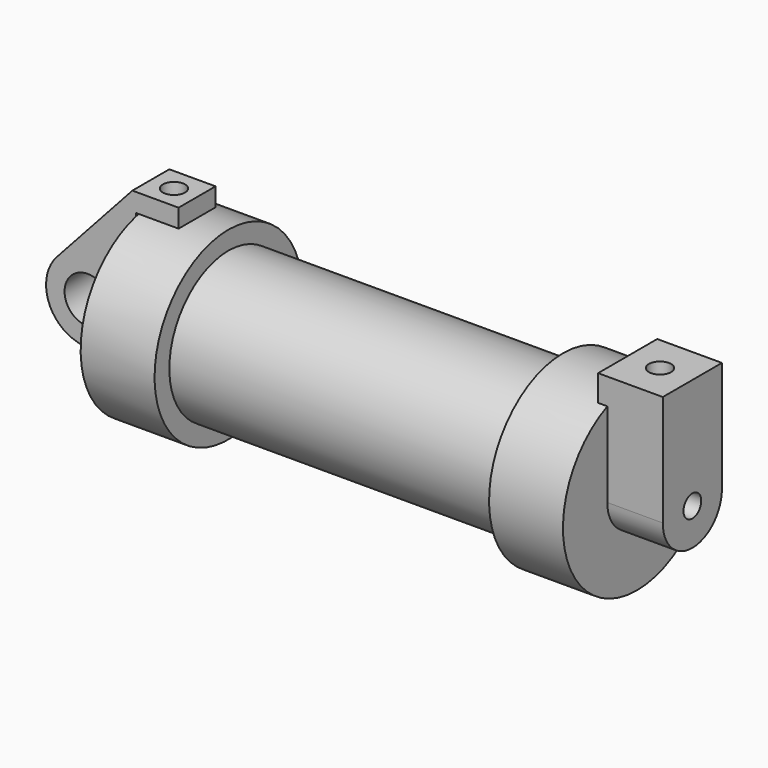
from build123d import *

# Parameters (mm, degrees)
F0_W          = 5.842
F0_H          = 12.7
F0_R          = 3.175
F2_DEPTH      = 3.175
F3_R          = 1.524
F4_DEPTH      = 7.62
F4_DEPTH_BACK = 1.27
F5_R          = 1.524
F6_DEPTH      = 10.414
F7_R          = 1.524
F8_DEPTH      = 17.78


with BuildPart() as f1:
    # F0 (on Front) → F1 (revolve)
    with BuildSketch(Plane.XZ):
        Polygon((5.842, 12.7), (5.842, 0), (66.294, 0), (66.294, 12.7), (56.134, 12.7), (56.134, 10.16), (10.16, 10.16), (10.16, 12.7), align=None)
        with Locations((2.921, 6.35)):
            Rectangle(F0_W, F0_H)
    revolve(axis=Axis((33.147, 0, 0), (-1, 0, 0)))

    # F3 (on face) → F4 (join, two sides)
    with BuildSketch(Plane.YZ.offset(66.294)) as f4_sk:
        with BuildLine():
            ThreePointArc((-5.08, 0), (0, -5.08), (5.08, 0))
            ThreePointArc((5.08, 0), (0, 5.08), (-5.08, 0))
        make_face()
        Circle(F3_R, mode=Mode.SUBTRACT)
        with BuildLine():
            ThreePointArc((-5.08, 11.6397422652), (0, 12.7), (5.08, 11.6397422652))
            Line((5.08, 11.6397422652), (5.08, 15.24))
            Line((5.08, 15.24), (-5.08, 15.24))
            Line((-5.08, 15.24), (-5.08, 11.6397422652))
        make_face()
        with BuildLine():
            ThreePointArc((-5.08, 0), (0, 5.08), (5.08, 0))
            Line((5.08, 0), (5.08, 11.6397422652))
            ThreePointArc((5.08, 11.6397422652), (0, 12.7), (-5.08, 11.6397422652))
            Line((-5.08, 11.6397422652), (-5.08, 0))
        make_face()
    extrude(amount=F4_DEPTH)
    extrude(f4_sk.sketch, amount=-F4_DEPTH_BACK)

    # F5 (on face) → F6 (cut)
    with BuildSketch(Plane.XY.offset(15.24)):
        with Locations((69.469, 0)):
            Circle(F5_R)
    extrude(amount=-F6_DEPTH, mode=Mode.SUBTRACT)


with BuildPart() as f2:
    # F0 (on Front) → F2 (new body, symmetric)
    with BuildSketch(Plane.XZ):
        with BuildLine():
            Line((5.842, 0), (0, 0))
            Line((0, 0), (-0.9398, 0))
            ThreePointArc((-0.9398, 0), (-3.1957909266, -4.5493385486), (-8.1826630726, -5.5069827884))
            Line((-8.1826630726, -5.5069827884), (5.842, -9.398))
            Line((5.842, -9.398), (5.842, 0))
        make_face()
        with BuildLine():
            Line((-0.9398, 0), (0, 0))
            Line((0, 0), (0, 12.7))
            Line((0, 12.7), (5.842, 12.7))
            Line((5.842, 12.7), (5.842, 15.24))
            Line((5.842, 15.24), (-0.508, 15.24))
            Line((-0.508, 15.24), (-10.8806298187, 3.8475430269))
            ThreePointArc((-10.8806298187, 3.8475430269), (-4.5919612295, 5.3297205562), (-0.9398, 0))
        make_face()
        with BuildLine():
            ThreePointArc((-8.1826630726, -5.5069827884), (-3.1957909266, -4.5493385486), (-0.9398, 0))
            ThreePointArc((-0.9398, 0), (-4.5919612295, 5.3297205562), (-10.8806298187, 3.8475430269))
            ThreePointArc((-10.8806298187, 3.8475430269), (-12.1459778134, -1.5837270034), (-8.1826630726, -5.5069827884))
        make_face()
        with Locations((-6.6548, 0)):
            Circle(F0_R, mode=Mode.SUBTRACT)
    extrude(amount=F2_DEPTH, both=True)

    # F7 (on face) → F8 (cut)
    with BuildSketch(Plane.XY.offset(15.24)):
        with Locations((2.667, 0)):
            Circle(F7_R)
    extrude(amount=-F8_DEPTH, mode=Mode.SUBTRACT)


solid = Compound([f1.part, f2.part])
